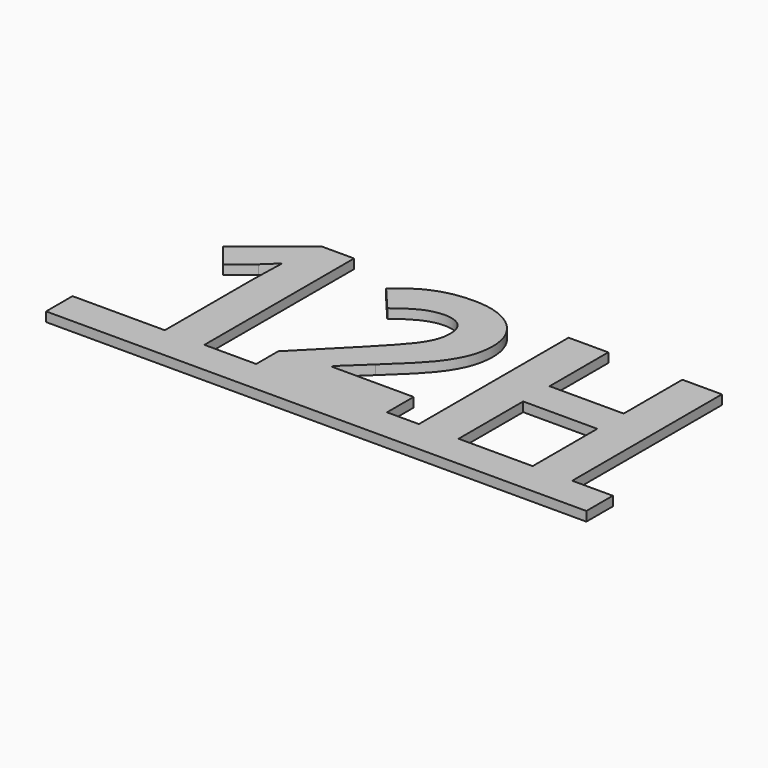
from build123d import *

# Parameters (mm, degrees)
F0_TEXT_SIZE = 1411.1111111111
F1_DEPTH     = 50.8


# Not quite as in the source:
# - a feature names something its author has since deleted; it is built from what else it names
# - Text() gives the source's letters only with a copy of the font that has no kerning and outlines rounded to 1/6400 em; it was checked with that copy


with BuildPart() as f1:
    # F0 (on Top) → F1 (new body)
    with BuildSketch(Plane.XY):
        Polygon((-308.6898137331, 0), (-308.6898137331, -177.8), (2599.9629640447, -177.8), (2599.9629640447, 0), (2381.4612279336, 0), (2168.4716446002, 0), (1769.6122696002, 0), (1555.9612279336, 0), (1384.4230334891, 0), (680.1903946002, 0), (401.2754640447, 0), (188.2858807113, 0), align=None)
        with Locations((-181.6898137331, 0)):
            Text('12H', F0_TEXT_SIZE, font='Open Sans', font_style=FontStyle.BOLD, text_align=(TextAlign.LEFT, TextAlign.BOTTOM))
    extrude(amount=F1_DEPTH)


solid = f1.part
